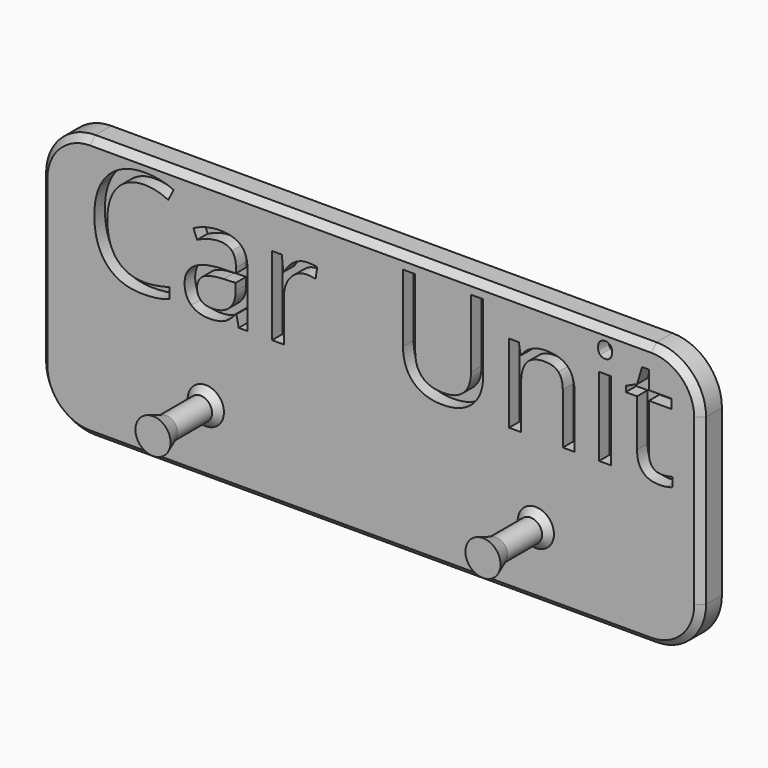
from build123d import *

# Parameters (mm, degrees)
F0_W         = 100
F0_H         = 40
F0_W_2       = 1.8020833333
F0_H_2       = 11.8923611111
F0_TEXT_SIZE = 22.2222222222
F1_DEPTH     = 2
F2_DEPTH     = 2
F3_R         = 1.75
F4_DEPTH     = 7.5
F4_FACE_R    = 1.75
F5_DEPTH     = 2.5
F5_TAPER     = -20
F6_R         = 7.5
F7_SIZE      = 1


# Not quite as in the source:
# - Text() gives the source's letters only with a copy of the font that has no kerning and outlines rounded to 1/6400 em; it was checked with that copy


with BuildPart() as f1:
    # F0 (on Front) → F1 (new body)
    with BuildSketch(Plane.XZ):
        Rectangle(F0_W, F0_H)
        with BuildLine():
            add(Edge.make_bspline(
                [(-30.6736111111, 15.5972222222), (-32.4756944444, 16.4409722222), (-34.2777777778, 16.4409722222)],
                knots=[0, 0, 0, 1, 1, 1], degree=2))
            add(Edge.make_bspline(
                [(-34.2777777778, 16.4409722222), (-36.8923611111, 16.4409722222), (-38.40625, 14.6996527778)],
                knots=[0, 0, 0, 1, 1, 1], degree=2))
            add(Edge.make_bspline(
                [(-38.40625, 14.6996527778), (-39.9201388889, 12.9583333333), (-39.9201388889, 9.9305555556)],
                knots=[0, 0, 0, 1, 1, 1], degree=2))
            add(Edge.make_bspline(
                [(-39.9201388889, 9.9305555556), (-39.9201388889, 6.8194444444), (-38.4600694444, 5.1197916667)],
                knots=[0, 0, 0, 1, 1, 1], degree=2))
            add(Edge.make_bspline(
                [(-38.4600694444, 5.1197916667), (-37, 3.4201388889), (-34.2986111111, 3.4201388889)],
                knots=[0, 0, 0, 1, 1, 1], degree=2))
            add(Edge.make_bspline(
                [(-34.2986111111, 3.4201388889), (-32.6388888889, 3.4201388889), (-30.5104166667, 4.0173611111)],
                knots=[0, 0, 0, 1, 1, 1], degree=2))
            Line((-30.5104166667, 4.0173611111), (-30.5104166667, 2.4027777778))
            add(Edge.make_bspline(
                [(-30.5104166667, 2.4027777778), (-32.1597222222, 1.78125), (-34.5798611111, 1.78125)],
                knots=[0, 0, 0, 1, 1, 1], degree=2))
            add(Edge.make_bspline(
                [(-34.5798611111, 1.78125), (-38.0833333333, 1.78125), (-39.9878472222, 3.9097222222)],
                knots=[0, 0, 0, 1, 1, 1], degree=2))
            add(Edge.make_bspline(
                [(-39.9878472222, 3.9097222222), (-41.8923611111, 6.0381944444), (-41.8923611111, 9.9548611111)],
                knots=[0, 0, 0, 1, 1, 1], degree=2))
            add(Edge.make_bspline(
                [(-41.8923611111, 9.9548611111), (-41.8923611111, 12.40625), (-40.9756944444, 14.25)],
                knots=[0, 0, 0, 1, 1, 1], degree=2))
            add(Edge.make_bspline(
                [(-40.9756944444, 14.25), (-40.0590277778, 16.09375), (-38.328125, 17.0920138889)],
                knots=[0, 0, 0, 1, 1, 1], degree=2))
            add(Edge.make_bspline(
                [(-38.328125, 17.0920138889), (-36.5972222222, 18.0902777778), (-34.2534722222, 18.0902777778)],
                knots=[0, 0, 0, 1, 1, 1], degree=2))
            add(Edge.make_bspline(
                [(-34.2534722222, 18.0902777778), (-31.7604166667, 18.0902777778), (-29.8923611111, 17.1805555556)],
                knots=[0, 0, 0, 1, 1, 1], degree=2))
            Line((-29.8923611111, 17.1805555556), (-30.6736111111, 15.5972222222))
        make_face(mode=Mode.SUBTRACT)
        with BuildLine():
            Line((-18.6701388889, 2), (-20.0069444444, 2))
            Line((-20.0069444444, 2), (-20.3645833333, 3.6944444444))
            Line((-20.3645833333, 3.6944444444), (-20.4513888889, 3.6944444444))
            add(Edge.make_bspline(
                [(-20.4513888889, 3.6944444444), (-21.3402777778, 2.5763888889), (-22.2239583333, 2.1788194444)],
                knots=[0, 0, 0, 1, 1, 1], degree=2))
            add(Edge.make_bspline(
                [(-22.2239583333, 2.1788194444), (-23.1076388889, 1.78125), (-24.4340277778, 1.78125)],
                knots=[0, 0, 0, 1, 1, 1], degree=2))
            add(Edge.make_bspline(
                [(-24.4340277778, 1.78125), (-26.2013888889, 1.78125), (-27.2048611111, 2.6944444444)],
                knots=[0, 0, 0, 1, 1, 1], degree=2))
            add(Edge.make_bspline(
                [(-27.2048611111, 2.6944444444), (-28.2083333333, 3.6076388889), (-28.2083333333, 5.2881944444)],
                knots=[0, 0, 0, 1, 1, 1], degree=2))
            add(Edge.make_bspline(
                [(-28.2083333333, 5.2881944444), (-28.2083333333, 8.8888888889), (-22.4479166667, 9.0625)],
                knots=[0, 0, 0, 1, 1, 1], degree=2))
            Line((-22.4479166667, 9.0625), (-20.4305555556, 9.1284722222))
            Line((-20.4305555556, 9.1284722222), (-20.4305555556, 9.8680555556))
            add(Edge.make_bspline(
                [(-20.4305555556, 9.8680555556), (-20.4305555556, 11.2673611111), (-21.03125, 11.9340277778)],
                knots=[0, 0, 0, 1, 1, 1], degree=2))
            add(Edge.make_bspline(
                [(-21.03125, 11.9340277778), (-21.6319444444, 12.6006944444), (-22.9583333333, 12.6006944444)],
                knots=[0, 0, 0, 1, 1, 1], degree=2))
            add(Edge.make_bspline(
                [(-22.9583333333, 12.6006944444), (-24.4444444444, 12.6006944444), (-26.3194444444, 11.6909722222)],
                knots=[0, 0, 0, 1, 1, 1], degree=2))
            Line((-26.3194444444, 11.6909722222), (-26.875, 13.0694444444))
            add(Edge.make_bspline(
                [(-26.875, 13.0694444444), (-25.9965277778, 13.5451388889), (-24.9496527778, 13.8159722222)],
                knots=[0, 0, 0, 1, 1, 1], degree=2))
            add(Edge.make_bspline(
                [(-24.9496527778, 13.8159722222), (-23.9027777778, 14.0868055556), (-22.8472222222, 14.0868055556)],
                knots=[0, 0, 0, 1, 1, 1], degree=2))
            add(Edge.make_bspline(
                [(-22.8472222222, 14.0868055556), (-20.7222222222, 14.0868055556), (-19.6961805556, 13.1440972222)],
                knots=[0, 0, 0, 1, 1, 1], degree=2))
            add(Edge.make_bspline(
                [(-19.6961805556, 13.1440972222), (-18.6701388889, 12.2013888889), (-18.6701388889, 10.1180555556)],
                knots=[0, 0, 0, 1, 1, 1], degree=2))
            Line((-18.6701388889, 10.1180555556), (-18.6701388889, 2))
        make_face(mode=Mode.SUBTRACT)
        with BuildLine():
            add(Edge.make_bspline(
                [(-11.5868055556, 13.4809027778), (-10.6527777778, 14.1111111111), (-9.5347222222, 14.1111111111)],
                knots=[0, 0, 0, 1, 1, 1], degree=2))
            add(Edge.make_bspline(
                [(-9.5347222222, 14.1111111111), (-8.7430555556, 14.1111111111), (-8.1145833333, 13.9791666667)],
                knots=[0, 0, 0, 1, 1, 1], degree=2))
            Line((-8.1145833333, 13.9791666667), (-8.3645833333, 12.3090277778))
            add(Edge.make_bspline(
                [(-8.3645833333, 12.3090277778), (-9.1006944444, 12.4722222222), (-9.6666666667, 12.4722222222)],
                knots=[0, 0, 0, 1, 1, 1], degree=2))
            add(Edge.make_bspline(
                [(-9.6666666667, 12.4722222222), (-11.1111111111, 12.4722222222), (-12.1354166667, 11.3003472222)],
                knots=[0, 0, 0, 1, 1, 1], degree=2))
            add(Edge.make_bspline(
                [(-12.1354166667, 11.3003472222), (-13.1597222222, 10.1284722222), (-13.1597222222, 8.3819444444)],
                knots=[0, 0, 0, 1, 1, 1], degree=2))
            Line((-13.1597222222, 8.3819444444), (-13.1597222222, 2))
            Line((-13.1597222222, 2), (-14.9618055556, 2))
            Line((-14.9618055556, 2), (-14.9618055556, 13.8923611111))
            Line((-14.9618055556, 13.8923611111), (-13.4756944444, 13.8923611111))
            Line((-13.4756944444, 13.8923611111), (-13.2673611111, 11.6909722222))
            Line((-13.2673611111, 11.6909722222), (-13.1805555556, 11.6909722222))
            add(Edge.make_bspline(
                [(-13.1805555556, 11.6909722222), (-12.5208333333, 12.8506944444), (-11.5868055556, 13.4809027778)],
                knots=[0, 0, 0, 1, 1, 1], degree=2))
        make_face(mode=Mode.SUBTRACT)
        with BuildLine():
            Line((15.1790277778, 17.8645833333), (17.0227777778, 17.8645833333))
            Line((17.0227777778, 17.8645833333), (17.0227777778, 7.6006944444))
            add(Edge.make_bspline(
                [(17.0227777778, 7.6006944444), (17.0227777778, 4.8854166667), (15.3838888889, 3.3333333333)],
                knots=[0, 0, 0, 1, 1, 1], degree=2))
            add(Edge.make_bspline(
                [(15.3838888889, 3.3333333333), (13.745, 1.78125), (10.8804166667, 1.78125)],
                knots=[0, 0, 0, 1, 1, 1], degree=2))
            add(Edge.make_bspline(
                [(10.8804166667, 1.78125), (8.0158333333, 1.78125), (6.448125, 3.3454861111)],
                knots=[0, 0, 0, 1, 1, 1], degree=2))
            add(Edge.make_bspline(
                [(6.448125, 3.3454861111), (4.8804166667, 4.9097222222), (4.8804166667, 7.6423611111)],
                knots=[0, 0, 0, 1, 1, 1], degree=2))
            Line((4.8804166667, 7.6423611111), (4.8804166667, 17.8645833333))
            Line((4.8804166667, 17.8645833333), (6.7276388889, 17.8645833333))
            Line((6.7276388889, 17.8645833333), (6.7276388889, 7.5138888889))
            add(Edge.make_bspline(
                [(6.7276388889, 7.5138888889), (6.7276388889, 5.5277777778), (7.8127083333, 4.4635416667)],
                knots=[0, 0, 0, 1, 1, 1], degree=2))
            add(Edge.make_bspline(
                [(7.8127083333, 4.4635416667), (8.8977777778, 3.3993055556), (11.0019444444, 3.3993055556)],
                knots=[0, 0, 0, 1, 1, 1], degree=2))
            add(Edge.make_bspline(
                [(11.0019444444, 3.3993055556), (13.0088888889, 3.3993055556), (14.0939583333, 4.46875)],
                knots=[0, 0, 0, 1, 1, 1], degree=2))
            add(Edge.make_bspline(
                [(14.0939583333, 4.46875), (15.1790277778, 5.5381944444), (15.1790277778, 7.5347222222)],
                knots=[0, 0, 0, 1, 1, 1], degree=2))
            Line((15.1790277778, 7.5347222222), (15.1790277778, 17.8645833333))
        make_face(mode=Mode.SUBTRACT)
        with BuildLine():
            Line((30.8908333333, 2), (29.08875, 2))
            Line((29.08875, 2), (29.08875, 9.6944444444))
            add(Edge.make_bspline(
                [(29.08875, 9.6944444444), (29.08875, 11.1458333333), (28.4272916667, 11.8628472222)],
                knots=[0, 0, 0, 1, 1, 1], degree=2))
            add(Edge.make_bspline(
                [(28.4272916667, 11.8628472222), (27.7658333333, 12.5798611111), (26.3526388889, 12.5798611111)],
                knots=[0, 0, 0, 1, 1, 1], degree=2))
            add(Edge.make_bspline(
                [(26.3526388889, 12.5798611111), (24.4880555556, 12.5798611111), (23.62, 11.5711805556)],
                knots=[0, 0, 0, 1, 1, 1], degree=2))
            add(Edge.make_bspline(
                [(23.62, 11.5711805556), (22.7519444444, 10.5625), (22.7519444444, 8.2395833333)],
                knots=[0, 0, 0, 1, 1, 1], degree=2))
            Line((22.7519444444, 8.2395833333), (22.7519444444, 2))
            Line((22.7519444444, 2), (20.9498611111, 2))
            Line((20.9498611111, 2), (20.9498611111, 13.8923611111))
            Line((20.9498611111, 13.8923611111), (22.4151388889, 13.8923611111))
            Line((22.4151388889, 13.8923611111), (22.7068055556, 12.2638888889))
            Line((22.7068055556, 12.2638888889), (22.7936111111, 12.2638888889))
            add(Edge.make_bspline(
                [(22.7936111111, 12.2638888889), (23.3491666667, 13.1423611111), (24.3474305556, 13.6267361111)],
                knots=[0, 0, 0, 1, 1, 1], degree=2))
            add(Edge.make_bspline(
                [(24.3474305556, 13.6267361111), (25.3456944444, 14.1111111111), (26.5713888889, 14.1111111111)],
                knots=[0, 0, 0, 1, 1, 1], degree=2))
            add(Edge.make_bspline(
                [(26.5713888889, 14.1111111111), (28.7206944444, 14.1111111111), (29.8057638889, 13.0746527778)],
                knots=[0, 0, 0, 1, 1, 1], degree=2))
            add(Edge.make_bspline(
                [(29.8057638889, 13.0746527778), (30.8908333333, 12.0381944444), (30.8908333333, 9.7569444444)],
                knots=[0, 0, 0, 1, 1, 1], degree=2))
            Line((30.8908333333, 9.7569444444), (30.8908333333, 2))
        make_face(mode=Mode.SUBTRACT)
        with Locations((35.4897916667, 7.9461805556)):
            Rectangle(F0_W_2, F0_H_2, mode=Mode.SUBTRACT)
        with BuildLine():
            add(Edge.make_bspline(
                [(42.65125, 3.8454861111), (43.1616666667, 3.2708333333), (44.0505555556, 3.2708333333)],
                knots=[0, 0, 0, 1, 1, 1], degree=2))
            add(Edge.make_bspline(
                [(44.0505555556, 3.2708333333), (44.5297222222, 3.2708333333), (44.9741666667, 3.3402777778)],
                knots=[0, 0, 0, 1, 1, 1], degree=2))
            add(Edge.make_bspline(
                [(44.9741666667, 3.3402777778), (45.4186111111, 3.4097222222), (45.6790277778, 3.4861111111)],
                knots=[0, 0, 0, 1, 1, 1], degree=2))
            Line((45.6790277778, 3.4861111111), (45.6790277778, 2.1076388889))
            add(Edge.make_bspline(
                [(45.6790277778, 2.1076388889), (45.3873611111, 1.96875), (44.8179166667, 1.875)],
                knots=[0, 0, 0, 1, 1, 1], degree=2))
            add(Edge.make_bspline(
                [(44.8179166667, 1.875), (44.2484722222, 1.78125), (43.7901388889, 1.78125)],
                knots=[0, 0, 0, 1, 1, 1], degree=2))
            add(Edge.make_bspline(
                [(43.7901388889, 1.78125), (40.3422222222, 1.78125), (40.3422222222, 5.4166666667)],
                knots=[0, 0, 0, 1, 1, 1], degree=2))
            Line((40.3422222222, 5.4166666667), (40.3422222222, 12.4930555556))
            Line((40.3422222222, 12.4930555556), (38.6373611111, 12.4930555556))
            Line((38.6373611111, 12.4930555556), (38.6373611111, 13.3611111111))
            Line((38.6373611111, 13.3611111111), (40.3422222222, 14.1111111111))
            Line((40.3422222222, 14.1111111111), (41.0991666667, 16.6493055556))
            Line((41.0991666667, 16.6493055556), (42.1408333333, 16.6493055556))
            Line((42.1408333333, 16.6493055556), (42.1408333333, 13.8923611111))
            Line((42.1408333333, 13.8923611111), (45.5922222222, 13.8923611111))
            Line((45.5922222222, 13.8923611111), (45.5922222222, 12.4930555556))
            Line((45.5922222222, 12.4930555556), (42.1408333333, 12.4930555556))
            Line((42.1408333333, 12.4930555556), (42.1408333333, 5.4930555556))
            add(Edge.make_bspline(
                [(42.1408333333, 5.4930555556), (42.1408333333, 4.4201388889), (42.65125, 3.8454861111)],
                knots=[0, 0, 0, 1, 1, 1], degree=2))
        make_face(mode=Mode.SUBTRACT)
        with BuildLine():
            add(Edge.make_bspline(
                [(34.7397916667, 16.2083333333), (34.4359722222, 16.5069444444), (34.4359722222, 17.1145833333)],
                knots=[0, 0, 0, 1, 1, 1], degree=2))
            add(Edge.make_bspline(
                [(34.4359722222, 17.1145833333), (34.4359722222, 17.7326388889), (34.7397916667, 18.0208333333)],
                knots=[0, 0, 0, 1, 1, 1], degree=2))
            add(Edge.make_bspline(
                [(34.7397916667, 18.0208333333), (35.0436111111, 18.3090277778), (35.5019444444, 18.3090277778)],
                knots=[0, 0, 0, 1, 1, 1], degree=2))
            add(Edge.make_bspline(
                [(35.5019444444, 18.3090277778), (35.9359722222, 18.3090277778), (36.2502083333, 18.015625)],
                knots=[0, 0, 0, 1, 1, 1], degree=2))
            add(Edge.make_bspline(
                [(36.2502083333, 18.015625), (36.5644444444, 17.7222222222), (36.5644444444, 17.1145833333)],
                knots=[0, 0, 0, 1, 1, 1], degree=2))
            add(Edge.make_bspline(
                [(36.5644444444, 17.1145833333), (36.5644444444, 16.5069444444), (36.2502083333, 16.2083333333)],
                knots=[0, 0, 0, 1, 1, 1], degree=2))
            add(Edge.make_bspline(
                [(36.2502083333, 16.2083333333), (35.9359722222, 15.9097222222), (35.5019444444, 15.9097222222)],
                knots=[0, 0, 0, 1, 1, 1], degree=2))
            add(Edge.make_bspline(
                [(35.5019444444, 15.9097222222), (35.0436111111, 15.9097222222), (34.7397916667, 16.2083333333)],
                knots=[0, 0, 0, 1, 1, 1], degree=2))
        make_face(mode=Mode.SUBTRACT)
        with Locations((-43.25, 2)):
            Text('Car', F0_TEXT_SIZE, font='Open Sans', text_align=(TextAlign.LEFT, TextAlign.BOTTOM))
        with BuildLine():
            add(Edge.make_bspline(
                [(-25.7291666667, 3.7795138889), (-25.1388888889, 3.2708333333), (-24.0763888889, 3.2708333333)],
                knots=[0, 0, 0, 1, 1, 1], degree=2))
            add(Edge.make_bspline(
                [(-24.0763888889, 3.2708333333), (-22.3923611111, 3.2708333333), (-21.4322916667, 4.1927083333)],
                knots=[0, 0, 0, 1, 1, 1], degree=2))
            add(Edge.make_bspline(
                [(-21.4322916667, 4.1927083333), (-20.4722222222, 5.1145833333), (-20.4722222222, 6.7743055556)],
                knots=[0, 0, 0, 1, 1, 1], degree=2))
            Line((-20.4722222222, 6.7743055556), (-20.4722222222, 7.8472222222))
            Line((-20.4722222222, 7.8472222222), (-22.2743055556, 7.7743055556))
            add(Edge.make_bspline(
                [(-22.2743055556, 7.7743055556), (-24.4236111111, 7.6979166667), (-25.3715277778, 7.1059027778)],
                knots=[0, 0, 0, 1, 1, 1], degree=2))
            add(Edge.make_bspline(
                [(-25.3715277778, 7.1059027778), (-26.3194444444, 6.5138888889), (-26.3194444444, 5.2673611111)],
                knots=[0, 0, 0, 1, 1, 1], degree=2))
            add(Edge.make_bspline(
                [(-26.3194444444, 5.2673611111), (-26.3194444444, 4.2881944444), (-25.7291666667, 3.7795138889)],
                knots=[0, 0, 0, 1, 1, 1], degree=2))
        make_face()
        with Locations((2.8630555556, 2)):
            Text('Unit', F0_TEXT_SIZE, font='Open Sans', text_align=(TextAlign.LEFT, TextAlign.BOTTOM))
    extrude(amount=-F1_DEPTH)

    # F0 (on Front) → F2 (join)
    with BuildSketch(Plane.XZ):
        Rectangle(F0_W, F0_H)
        with BuildLine():
            add(Edge.make_bspline(
                [(-30.6736111111, 15.5972222222), (-32.4756944444, 16.4409722222), (-34.2777777778, 16.4409722222)],
                knots=[0, 0, 0, 1, 1, 1], degree=2))
            add(Edge.make_bspline(
                [(-34.2777777778, 16.4409722222), (-36.8923611111, 16.4409722222), (-38.40625, 14.6996527778)],
                knots=[0, 0, 0, 1, 1, 1], degree=2))
            add(Edge.make_bspline(
                [(-38.40625, 14.6996527778), (-39.9201388889, 12.9583333333), (-39.9201388889, 9.9305555556)],
                knots=[0, 0, 0, 1, 1, 1], degree=2))
            add(Edge.make_bspline(
                [(-39.9201388889, 9.9305555556), (-39.9201388889, 6.8194444444), (-38.4600694444, 5.1197916667)],
                knots=[0, 0, 0, 1, 1, 1], degree=2))
            add(Edge.make_bspline(
                [(-38.4600694444, 5.1197916667), (-37, 3.4201388889), (-34.2986111111, 3.4201388889)],
                knots=[0, 0, 0, 1, 1, 1], degree=2))
            add(Edge.make_bspline(
                [(-34.2986111111, 3.4201388889), (-32.6388888889, 3.4201388889), (-30.5104166667, 4.0173611111)],
                knots=[0, 0, 0, 1, 1, 1], degree=2))
            Line((-30.5104166667, 4.0173611111), (-30.5104166667, 2.4027777778))
            add(Edge.make_bspline(
                [(-30.5104166667, 2.4027777778), (-32.1597222222, 1.78125), (-34.5798611111, 1.78125)],
                knots=[0, 0, 0, 1, 1, 1], degree=2))
            add(Edge.make_bspline(
                [(-34.5798611111, 1.78125), (-38.0833333333, 1.78125), (-39.9878472222, 3.9097222222)],
                knots=[0, 0, 0, 1, 1, 1], degree=2))
            add(Edge.make_bspline(
                [(-39.9878472222, 3.9097222222), (-41.8923611111, 6.0381944444), (-41.8923611111, 9.9548611111)],
                knots=[0, 0, 0, 1, 1, 1], degree=2))
            add(Edge.make_bspline(
                [(-41.8923611111, 9.9548611111), (-41.8923611111, 12.40625), (-40.9756944444, 14.25)],
                knots=[0, 0, 0, 1, 1, 1], degree=2))
            add(Edge.make_bspline(
                [(-40.9756944444, 14.25), (-40.0590277778, 16.09375), (-38.328125, 17.0920138889)],
                knots=[0, 0, 0, 1, 1, 1], degree=2))
            add(Edge.make_bspline(
                [(-38.328125, 17.0920138889), (-36.5972222222, 18.0902777778), (-34.2534722222, 18.0902777778)],
                knots=[0, 0, 0, 1, 1, 1], degree=2))
            add(Edge.make_bspline(
                [(-34.2534722222, 18.0902777778), (-31.7604166667, 18.0902777778), (-29.8923611111, 17.1805555556)],
                knots=[0, 0, 0, 1, 1, 1], degree=2))
            Line((-29.8923611111, 17.1805555556), (-30.6736111111, 15.5972222222))
        make_face(mode=Mode.SUBTRACT)
        with BuildLine():
            Line((-18.6701388889, 2), (-20.0069444444, 2))
            Line((-20.0069444444, 2), (-20.3645833333, 3.6944444444))
            Line((-20.3645833333, 3.6944444444), (-20.4513888889, 3.6944444444))
            add(Edge.make_bspline(
                [(-20.4513888889, 3.6944444444), (-21.3402777778, 2.5763888889), (-22.2239583333, 2.1788194444)],
                knots=[0, 0, 0, 1, 1, 1], degree=2))
            add(Edge.make_bspline(
                [(-22.2239583333, 2.1788194444), (-23.1076388889, 1.78125), (-24.4340277778, 1.78125)],
                knots=[0, 0, 0, 1, 1, 1], degree=2))
            add(Edge.make_bspline(
                [(-24.4340277778, 1.78125), (-26.2013888889, 1.78125), (-27.2048611111, 2.6944444444)],
                knots=[0, 0, 0, 1, 1, 1], degree=2))
            add(Edge.make_bspline(
                [(-27.2048611111, 2.6944444444), (-28.2083333333, 3.6076388889), (-28.2083333333, 5.2881944444)],
                knots=[0, 0, 0, 1, 1, 1], degree=2))
            add(Edge.make_bspline(
                [(-28.2083333333, 5.2881944444), (-28.2083333333, 8.8888888889), (-22.4479166667, 9.0625)],
                knots=[0, 0, 0, 1, 1, 1], degree=2))
            Line((-22.4479166667, 9.0625), (-20.4305555556, 9.1284722222))
            Line((-20.4305555556, 9.1284722222), (-20.4305555556, 9.8680555556))
            add(Edge.make_bspline(
                [(-20.4305555556, 9.8680555556), (-20.4305555556, 11.2673611111), (-21.03125, 11.9340277778)],
                knots=[0, 0, 0, 1, 1, 1], degree=2))
            add(Edge.make_bspline(
                [(-21.03125, 11.9340277778), (-21.6319444444, 12.6006944444), (-22.9583333333, 12.6006944444)],
                knots=[0, 0, 0, 1, 1, 1], degree=2))
            add(Edge.make_bspline(
                [(-22.9583333333, 12.6006944444), (-24.4444444444, 12.6006944444), (-26.3194444444, 11.6909722222)],
                knots=[0, 0, 0, 1, 1, 1], degree=2))
            Line((-26.3194444444, 11.6909722222), (-26.875, 13.0694444444))
            add(Edge.make_bspline(
                [(-26.875, 13.0694444444), (-25.9965277778, 13.5451388889), (-24.9496527778, 13.8159722222)],
                knots=[0, 0, 0, 1, 1, 1], degree=2))
            add(Edge.make_bspline(
                [(-24.9496527778, 13.8159722222), (-23.9027777778, 14.0868055556), (-22.8472222222, 14.0868055556)],
                knots=[0, 0, 0, 1, 1, 1], degree=2))
            add(Edge.make_bspline(
                [(-22.8472222222, 14.0868055556), (-20.7222222222, 14.0868055556), (-19.6961805556, 13.1440972222)],
                knots=[0, 0, 0, 1, 1, 1], degree=2))
            add(Edge.make_bspline(
                [(-19.6961805556, 13.1440972222), (-18.6701388889, 12.2013888889), (-18.6701388889, 10.1180555556)],
                knots=[0, 0, 0, 1, 1, 1], degree=2))
            Line((-18.6701388889, 10.1180555556), (-18.6701388889, 2))
        make_face(mode=Mode.SUBTRACT)
        with BuildLine():
            add(Edge.make_bspline(
                [(-11.5868055556, 13.4809027778), (-10.6527777778, 14.1111111111), (-9.5347222222, 14.1111111111)],
                knots=[0, 0, 0, 1, 1, 1], degree=2))
            add(Edge.make_bspline(
                [(-9.5347222222, 14.1111111111), (-8.7430555556, 14.1111111111), (-8.1145833333, 13.9791666667)],
                knots=[0, 0, 0, 1, 1, 1], degree=2))
            Line((-8.1145833333, 13.9791666667), (-8.3645833333, 12.3090277778))
            add(Edge.make_bspline(
                [(-8.3645833333, 12.3090277778), (-9.1006944444, 12.4722222222), (-9.6666666667, 12.4722222222)],
                knots=[0, 0, 0, 1, 1, 1], degree=2))
            add(Edge.make_bspline(
                [(-9.6666666667, 12.4722222222), (-11.1111111111, 12.4722222222), (-12.1354166667, 11.3003472222)],
                knots=[0, 0, 0, 1, 1, 1], degree=2))
            add(Edge.make_bspline(
                [(-12.1354166667, 11.3003472222), (-13.1597222222, 10.1284722222), (-13.1597222222, 8.3819444444)],
                knots=[0, 0, 0, 1, 1, 1], degree=2))
            Line((-13.1597222222, 8.3819444444), (-13.1597222222, 2))
            Line((-13.1597222222, 2), (-14.9618055556, 2))
            Line((-14.9618055556, 2), (-14.9618055556, 13.8923611111))
            Line((-14.9618055556, 13.8923611111), (-13.4756944444, 13.8923611111))
            Line((-13.4756944444, 13.8923611111), (-13.2673611111, 11.6909722222))
            Line((-13.2673611111, 11.6909722222), (-13.1805555556, 11.6909722222))
            add(Edge.make_bspline(
                [(-13.1805555556, 11.6909722222), (-12.5208333333, 12.8506944444), (-11.5868055556, 13.4809027778)],
                knots=[0, 0, 0, 1, 1, 1], degree=2))
        make_face(mode=Mode.SUBTRACT)
        with BuildLine():
            Line((15.1790277778, 17.8645833333), (17.0227777778, 17.8645833333))
            Line((17.0227777778, 17.8645833333), (17.0227777778, 7.6006944444))
            add(Edge.make_bspline(
                [(17.0227777778, 7.6006944444), (17.0227777778, 4.8854166667), (15.3838888889, 3.3333333333)],
                knots=[0, 0, 0, 1, 1, 1], degree=2))
            add(Edge.make_bspline(
                [(15.3838888889, 3.3333333333), (13.745, 1.78125), (10.8804166667, 1.78125)],
                knots=[0, 0, 0, 1, 1, 1], degree=2))
            add(Edge.make_bspline(
                [(10.8804166667, 1.78125), (8.0158333333, 1.78125), (6.448125, 3.3454861111)],
                knots=[0, 0, 0, 1, 1, 1], degree=2))
            add(Edge.make_bspline(
                [(6.448125, 3.3454861111), (4.8804166667, 4.9097222222), (4.8804166667, 7.6423611111)],
                knots=[0, 0, 0, 1, 1, 1], degree=2))
            Line((4.8804166667, 7.6423611111), (4.8804166667, 17.8645833333))
            Line((4.8804166667, 17.8645833333), (6.7276388889, 17.8645833333))
            Line((6.7276388889, 17.8645833333), (6.7276388889, 7.5138888889))
            add(Edge.make_bspline(
                [(6.7276388889, 7.5138888889), (6.7276388889, 5.5277777778), (7.8127083333, 4.4635416667)],
                knots=[0, 0, 0, 1, 1, 1], degree=2))
            add(Edge.make_bspline(
                [(7.8127083333, 4.4635416667), (8.8977777778, 3.3993055556), (11.0019444444, 3.3993055556)],
                knots=[0, 0, 0, 1, 1, 1], degree=2))
            add(Edge.make_bspline(
                [(11.0019444444, 3.3993055556), (13.0088888889, 3.3993055556), (14.0939583333, 4.46875)],
                knots=[0, 0, 0, 1, 1, 1], degree=2))
            add(Edge.make_bspline(
                [(14.0939583333, 4.46875), (15.1790277778, 5.5381944444), (15.1790277778, 7.5347222222)],
                knots=[0, 0, 0, 1, 1, 1], degree=2))
            Line((15.1790277778, 7.5347222222), (15.1790277778, 17.8645833333))
        make_face(mode=Mode.SUBTRACT)
        with BuildLine():
            Line((30.8908333333, 2), (29.08875, 2))
            Line((29.08875, 2), (29.08875, 9.6944444444))
            add(Edge.make_bspline(
                [(29.08875, 9.6944444444), (29.08875, 11.1458333333), (28.4272916667, 11.8628472222)],
                knots=[0, 0, 0, 1, 1, 1], degree=2))
            add(Edge.make_bspline(
                [(28.4272916667, 11.8628472222), (27.7658333333, 12.5798611111), (26.3526388889, 12.5798611111)],
                knots=[0, 0, 0, 1, 1, 1], degree=2))
            add(Edge.make_bspline(
                [(26.3526388889, 12.5798611111), (24.4880555556, 12.5798611111), (23.62, 11.5711805556)],
                knots=[0, 0, 0, 1, 1, 1], degree=2))
            add(Edge.make_bspline(
                [(23.62, 11.5711805556), (22.7519444444, 10.5625), (22.7519444444, 8.2395833333)],
                knots=[0, 0, 0, 1, 1, 1], degree=2))
            Line((22.7519444444, 8.2395833333), (22.7519444444, 2))
            Line((22.7519444444, 2), (20.9498611111, 2))
            Line((20.9498611111, 2), (20.9498611111, 13.8923611111))
            Line((20.9498611111, 13.8923611111), (22.4151388889, 13.8923611111))
            Line((22.4151388889, 13.8923611111), (22.7068055556, 12.2638888889))
            Line((22.7068055556, 12.2638888889), (22.7936111111, 12.2638888889))
            add(Edge.make_bspline(
                [(22.7936111111, 12.2638888889), (23.3491666667, 13.1423611111), (24.3474305556, 13.6267361111)],
                knots=[0, 0, 0, 1, 1, 1], degree=2))
            add(Edge.make_bspline(
                [(24.3474305556, 13.6267361111), (25.3456944444, 14.1111111111), (26.5713888889, 14.1111111111)],
                knots=[0, 0, 0, 1, 1, 1], degree=2))
            add(Edge.make_bspline(
                [(26.5713888889, 14.1111111111), (28.7206944444, 14.1111111111), (29.8057638889, 13.0746527778)],
                knots=[0, 0, 0, 1, 1, 1], degree=2))
            add(Edge.make_bspline(
                [(29.8057638889, 13.0746527778), (30.8908333333, 12.0381944444), (30.8908333333, 9.7569444444)],
                knots=[0, 0, 0, 1, 1, 1], degree=2))
            Line((30.8908333333, 9.7569444444), (30.8908333333, 2))
        make_face(mode=Mode.SUBTRACT)
        with Locations((35.4897916667, 7.9461805556)):
            Rectangle(F0_W_2, F0_H_2, mode=Mode.SUBTRACT)
        with BuildLine():
            add(Edge.make_bspline(
                [(42.65125, 3.8454861111), (43.1616666667, 3.2708333333), (44.0505555556, 3.2708333333)],
                knots=[0, 0, 0, 1, 1, 1], degree=2))
            add(Edge.make_bspline(
                [(44.0505555556, 3.2708333333), (44.5297222222, 3.2708333333), (44.9741666667, 3.3402777778)],
                knots=[0, 0, 0, 1, 1, 1], degree=2))
            add(Edge.make_bspline(
                [(44.9741666667, 3.3402777778), (45.4186111111, 3.4097222222), (45.6790277778, 3.4861111111)],
                knots=[0, 0, 0, 1, 1, 1], degree=2))
            Line((45.6790277778, 3.4861111111), (45.6790277778, 2.1076388889))
            add(Edge.make_bspline(
                [(45.6790277778, 2.1076388889), (45.3873611111, 1.96875), (44.8179166667, 1.875)],
                knots=[0, 0, 0, 1, 1, 1], degree=2))
            add(Edge.make_bspline(
                [(44.8179166667, 1.875), (44.2484722222, 1.78125), (43.7901388889, 1.78125)],
                knots=[0, 0, 0, 1, 1, 1], degree=2))
            add(Edge.make_bspline(
                [(43.7901388889, 1.78125), (40.3422222222, 1.78125), (40.3422222222, 5.4166666667)],
                knots=[0, 0, 0, 1, 1, 1], degree=2))
            Line((40.3422222222, 5.4166666667), (40.3422222222, 12.4930555556))
            Line((40.3422222222, 12.4930555556), (38.6373611111, 12.4930555556))
            Line((38.6373611111, 12.4930555556), (38.6373611111, 13.3611111111))
            Line((38.6373611111, 13.3611111111), (40.3422222222, 14.1111111111))
            Line((40.3422222222, 14.1111111111), (41.0991666667, 16.6493055556))
            Line((41.0991666667, 16.6493055556), (42.1408333333, 16.6493055556))
            Line((42.1408333333, 16.6493055556), (42.1408333333, 13.8923611111))
            Line((42.1408333333, 13.8923611111), (45.5922222222, 13.8923611111))
            Line((45.5922222222, 13.8923611111), (45.5922222222, 12.4930555556))
            Line((45.5922222222, 12.4930555556), (42.1408333333, 12.4930555556))
            Line((42.1408333333, 12.4930555556), (42.1408333333, 5.4930555556))
            add(Edge.make_bspline(
                [(42.1408333333, 5.4930555556), (42.1408333333, 4.4201388889), (42.65125, 3.8454861111)],
                knots=[0, 0, 0, 1, 1, 1], degree=2))
        make_face(mode=Mode.SUBTRACT)
        with BuildLine():
            add(Edge.make_bspline(
                [(34.7397916667, 16.2083333333), (34.4359722222, 16.5069444444), (34.4359722222, 17.1145833333)],
                knots=[0, 0, 0, 1, 1, 1], degree=2))
            add(Edge.make_bspline(
                [(34.4359722222, 17.1145833333), (34.4359722222, 17.7326388889), (34.7397916667, 18.0208333333)],
                knots=[0, 0, 0, 1, 1, 1], degree=2))
            add(Edge.make_bspline(
                [(34.7397916667, 18.0208333333), (35.0436111111, 18.3090277778), (35.5019444444, 18.3090277778)],
                knots=[0, 0, 0, 1, 1, 1], degree=2))
            add(Edge.make_bspline(
                [(35.5019444444, 18.3090277778), (35.9359722222, 18.3090277778), (36.2502083333, 18.015625)],
                knots=[0, 0, 0, 1, 1, 1], degree=2))
            add(Edge.make_bspline(
                [(36.2502083333, 18.015625), (36.5644444444, 17.7222222222), (36.5644444444, 17.1145833333)],
                knots=[0, 0, 0, 1, 1, 1], degree=2))
            add(Edge.make_bspline(
                [(36.5644444444, 17.1145833333), (36.5644444444, 16.5069444444), (36.2502083333, 16.2083333333)],
                knots=[0, 0, 0, 1, 1, 1], degree=2))
            add(Edge.make_bspline(
                [(36.2502083333, 16.2083333333), (35.9359722222, 15.9097222222), (35.5019444444, 15.9097222222)],
                knots=[0, 0, 0, 1, 1, 1], degree=2))
            add(Edge.make_bspline(
                [(35.5019444444, 15.9097222222), (35.0436111111, 15.9097222222), (34.7397916667, 16.2083333333)],
                knots=[0, 0, 0, 1, 1, 1], degree=2))
        make_face(mode=Mode.SUBTRACT)
        with BuildLine():
            add(Edge.make_bspline(
                [(-25.7291666667, 3.7795138889), (-25.1388888889, 3.2708333333), (-24.0763888889, 3.2708333333)],
                knots=[0, 0, 0, 1, 1, 1], degree=2))
            add(Edge.make_bspline(
                [(-24.0763888889, 3.2708333333), (-22.3923611111, 3.2708333333), (-21.4322916667, 4.1927083333)],
                knots=[0, 0, 0, 1, 1, 1], degree=2))
            add(Edge.make_bspline(
                [(-21.4322916667, 4.1927083333), (-20.4722222222, 5.1145833333), (-20.4722222222, 6.7743055556)],
                knots=[0, 0, 0, 1, 1, 1], degree=2))
            Line((-20.4722222222, 6.7743055556), (-20.4722222222, 7.8472222222))
            Line((-20.4722222222, 7.8472222222), (-22.2743055556, 7.7743055556))
            add(Edge.make_bspline(
                [(-22.2743055556, 7.7743055556), (-24.4236111111, 7.6979166667), (-25.3715277778, 7.1059027778)],
                knots=[0, 0, 0, 1, 1, 1], degree=2))
            add(Edge.make_bspline(
                [(-25.3715277778, 7.1059027778), (-26.3194444444, 6.5138888889), (-26.3194444444, 5.2673611111)],
                knots=[0, 0, 0, 1, 1, 1], degree=2))
            add(Edge.make_bspline(
                [(-26.3194444444, 5.2673611111), (-26.3194444444, 4.2881944444), (-25.7291666667, 3.7795138889)],
                knots=[0, 0, 0, 1, 1, 1], degree=2))
        make_face()
    extrude(amount=F2_DEPTH)

    # F3 (on face) → F4 (join)
    with BuildSketch(Plane.XZ.offset(2)):
        with Locations((-25, -10)):
            Circle(F3_R)
        with Locations((25, -10)):
            Circle(F3_R)
    extrude(amount=F4_DEPTH)

    # F4_face (on face) → F5 (join)
    with BuildSketch(Plane(origin=(-25, -9.5, -10), x_dir=(1, 0, 0), z_dir=(0, -1, 0))):
        Circle(F4_FACE_R)
        with Locations((50, 0)):
            Circle(F4_FACE_R)
    extrude(amount=F5_DEPTH, taper=F5_TAPER)

    # F6
    f6_edges = [f1.edges().sort_by_distance(p)[0] for p in [
        (-50, 0, 20),
        (50, 0, 20),
        (50, 0, -20),
        (-50, 0, -20),
    ]]
    fillet(f6_edges, radius=F6_R)

    # F7
    f7_edges = [f1.edges().sort_by_distance(p)[0] for p in [
        (-50, -2, 0),
        (-26.75, -2, -10),
        (23.25, -2, -10),
    ]]
    chamfer(f7_edges, length=F7_SIZE)


solid = f1.part
